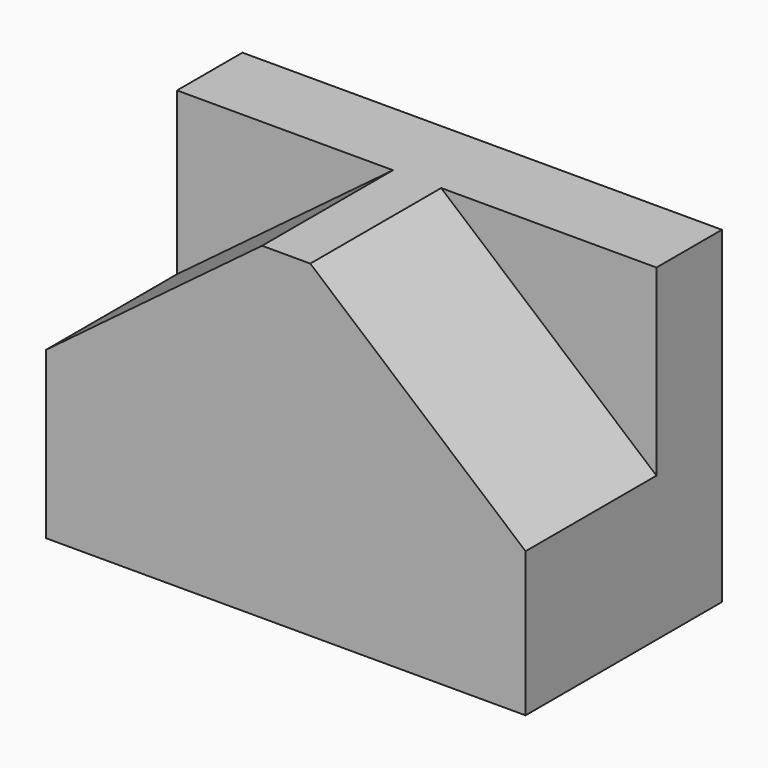
from build123d import *

# Parameters (mm, degrees)
F0_W     = 148.8501727581
F0_H     = 101.742612198
F1_DEPTH = 50.8
F3_DEPTH = 25.4
F5_DEPTH = 25.4


with BuildPart() as f1:
    # F0 (on Front) → F1 (new body)
    with BuildSketch(Plane.XZ):
        with Locations((-1.6997531056, 25.3749480471)):
            Rectangle(F0_W, F0_H)
    extrude(amount=F1_DEPTH)

    # F2 (on face) → F3 (cut)
    with BuildSketch(Plane.XZ.offset(50.8)):
        Polygon((-9.0788973585, 76.2462541461), (-76.1248394847, 76.2462541461), (-76.1248394847, 26.0104050889), align=None)
        Polygon((72.7253332734, 76.2462541461), (5.8954056378, 76.2462541461), (72.7253332734, 19.3677039224), align=None)
    extrude(amount=-F3_DEPTH, mode=Mode.SUBTRACT)

    # F1_face (on face) + F4 (on face) → F5 (join)
    with BuildSketch(Plane(origin=(-1.6997531056, -50.8, 25.3749480471), x_dir=(1, 0, 0), z_dir=(0, -1, 0))):
        Polygon((74.4250863791, -6.0072441247), (7.5951587435, 50.871306099), (-7.3791442529, 50.871306099), (-74.4250863791, 0.6354570418), (-74.4250863791, -50.871306099), (74.4250863791, -50.871306099), align=None)
    with BuildSketch(Plane.XZ.offset(50.8)):
        Polygon((72.7253332734, -25.4963580519), (72.7253332734, 19.3677039224), (5.8954056378, 76.2462541461), (-9.0788973585, 76.2462541461), (-76.1248394847, 26.0104050889), (-76.1248394847, -25.4963580519), align=None)
    extrude(amount=F5_DEPTH)


solid = f1.part
